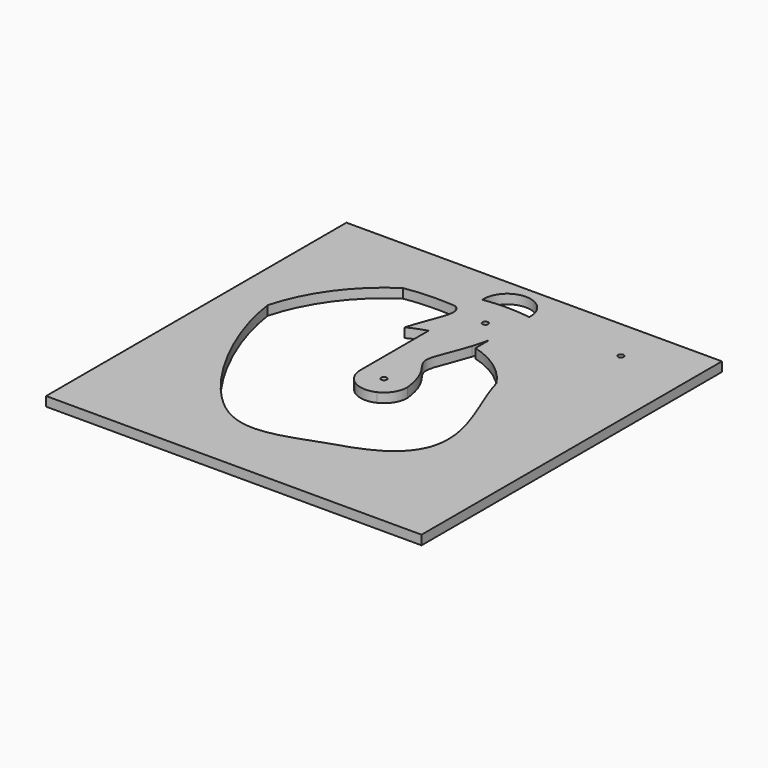
from build123d import *

# Parameters (mm, degrees)
F0_W     = 200
F0_H     = 200
F1_DEPTH = 5
F2_R     = 1.5
F3_DEPTH = 5.001
F4_R     = 1.5
F5_DEPTH = 5.001


# Not quite as in the source:
# - a feature names something its author has since deleted; it is built from what else it names


with BuildPart() as f1:
    # F0 (on Top) → F1 (new body)
    with BuildSketch(Plane.XY):
        Rectangle(F0_W, F0_H)
    extrude(amount=F1_DEPTH)

    # F2 (on face) → F3 (cut, through all)
    with BuildSketch(Plane.XY.offset(5)):
        Circle(F2_R)
        with Locations((0, -63.662)):
            Circle(F2_R)
        with Locations((64.1583176089, 77.5462182691)):
            Circle(F2_R)
        with Locations((-51.9230208324, 31.0114389966)):
            Circle(F2_R)
        with Locations((1.6717778053, 65.3690844774)):
            Circle(F2_R)
    extrude(amount=-F3_DEPTH, mode=Mode.SUBTRACT)

    # F4 (on face) → F5 (cut, through all)
    with BuildSketch(Plane.XY.offset(5)):
        with BuildLine():
            Line((-12.5, 0), (-12.5, 45.3072841826))
            ThreePointArc((-12.5, 45.3072841826), (-17.4301226021, 43.6484916816), (-22.1467463119, 41.4550555156))
            add(Edge.make_bspline(
                [(-22.1467463119, 41.4550555156), (-22.9092474685, 38.6087716354), (-26.7916480004, 19.492616055), (-18.2157949408, -4.2593218119), (-6.9475647742, -10.3914072054)],
                knots=[0.382428707, 0.382428707, 0.382428707, 0.382428707, 0.4580536444, 0.8659002673, 0.8659002673, 0.8659002673, 0.8659002673], degree=3))
            ThreePointArc((-6.9475647742, -10.3914072054), (-11.024848291, -5.8909014727), (-12.5, 0))
        make_face()
        with BuildLine():
            ThreePointArc((-44.8138332434, 68.6711027291), (-66.3187168056, 48.2268369402), (-79.1399512645, 21.4678390587))
            add(Edge.make_bspline(
                [(28.4173693508, -56.6046871245), (3.9913801126, -64.1205269264), (-32.503865236, -87.7373972459), (-75.0211054276, -9.8932929428), (-79.1399512645, 21.4678390587)],
                knots=[0, 0, 0, 0, 0.2921661902, 0.6142842516, 0.6142842516, 0.6142842516, 0.6142842516], degree=3))
            add(Edge.make_bspline(
                [(28.4173693508, -56.6046871245), (64.8528327163, -43.3941669474), (56.1975225425, -18.4447190671), (46.7037719975, 5.2685558936)],
                knots=[0, 0, 0, 0, 0.1772966077, 0.1772966077, 0.1772966077, 0.1772966077], degree=3))
            ThreePointArc((46.7037719975, 5.2685558936), (46.9258845622, 2.6384385644), (47, 0))
            ThreePointArc((47, 0), (-24.1671566733, -40.310650433), (-22.1467463119, 41.4550555156))
            add(Edge.make_bspline(
                [(-18.0183753353, 69.6594335387), (-10.4657655575, 66.5625813654), (-18.2908445233, 55.8484646377), (-22.1467463119, 41.4550555156)],
                knots=[0, 0, 0, 0, 0.382428707, 0.382428707, 0.382428707, 0.382428707], degree=3))
            add(Edge.make_bspline(
                [(-44.8138332434, 68.6711027291), (-36.4977633391, 70.1220717043), (-27.3217936199, 70.3416004143), (-18.0183753353, 69.6594335387)],
                knots=[0.898151434, 0.898151434, 0.898151434, 0.898151434, 1, 1, 1, 1], degree=3))
        make_face()
        with Locations((0, -63.662)):
            Circle(F4_R, mode=Mode.SUBTRACT)
        with Locations((-51.9230208324, 31.0114389966)):
            Circle(F4_R, mode=Mode.SUBTRACT)
        with BuildLine():
            add(Edge.make_bspline(
                [(46.7037719975, 5.2685558936), (43.8279453898, 12.4517304214), (40.8751841388, 19.5214746733), (39.0755044059, 26.1171391125)],
                knots=[0.1772966077, 0.1772966077, 0.1772966077, 0.1772966077, 0.2310029169, 0.2310029169, 0.2310029169, 0.2310029169], degree=3))
            ThreePointArc((39.0755044059, 26.1171391125), (27.5149701187, 38.1041522589), (12.5, 45.3072841826))
            Line((12.5, 45.3072841826), (12.5, 0))
            ThreePointArc((12.5, 0), (10.548673601, -6.7063764627), (5.3039223586, -11.318940216))
            ThreePointArc((5.3039223586, -11.318940216), (-0.9436468985, -12.4643303282), (-6.9475647742, -10.3914072054))
            add(Edge.make_bspline(
                [(-22.1467463119, 41.4550555156), (-22.9092474685, 38.6087716354), (-26.7916480004, 19.492616055), (-18.2157949408, -4.2593218119), (-6.9475647742, -10.3914072054)],
                knots=[0.382428707, 0.382428707, 0.382428707, 0.382428707, 0.4580536444, 0.8659002673, 0.8659002673, 0.8659002673, 0.8659002673], degree=3))
            ThreePointArc((-22.1467463119, 41.4550555156), (-24.1671566733, -40.310650433), (47, 0))
            ThreePointArc((47, 0), (46.9258845622, 2.6384385644), (46.7037719975, 5.2685558936))
        make_face()
        with BuildLine():
            Line((12.5, 0), (12.5, 45.3072841826))
            ThreePointArc((12.5, 45.3072841826), (11.372638641, 45.6033232379), (10.2382828633, 45.8713152636))
            add(Edge.make_bspline(
                [(12.5, 0), (10.6902167617, 15.518115425), (-2.0681567086, 20.0495964199), (6.7073533039, 34.5490943361), (10.2382828633, 45.8713152636)],
                knots=[0, 0, 0, 0, 0.4638904895, 0.8993636987, 0.8993636987, 0.8993636987, 0.8993636987], degree=3))
        make_face()
        with BuildLine():
            Line((12.5, 45.3072841826), (12.5, 54.4343143702))
            add(Edge.make_bspline(
                [(10.2382828633, 45.8713152636), (11.0542680571, 48.4878400289), (11.8318981736, 51.3340910932), (12.5, 54.4343143702)],
                knots=[0.8993636987, 0.8993636987, 0.8993636987, 0.8993636987, 1, 1, 1, 1], degree=3))
            ThreePointArc((10.2382828633, 45.8713152636), (11.372638641, 45.6033232379), (12.5, 45.3072841826))
        make_face()
        with BuildLine():
            Line((-12.5, 82), (-12.5, 81.0416559554))
            ThreePointArc((-12.5, 81.0416559554), (-6.2683415531, 81.7600629536), (0, 82))
            ThreePointArc((0, 82), (6.2683415531, 81.7600629536), (12.5, 81.0416559554))
            Line((12.5, 81.0416559554), (12.5, 82))
            ThreePointArc((12.5, 82), (0, 94.5), (-12.5, 82))
        make_face()
    extrude(amount=-F5_DEPTH, mode=Mode.SUBTRACT)


solid = f1.part
